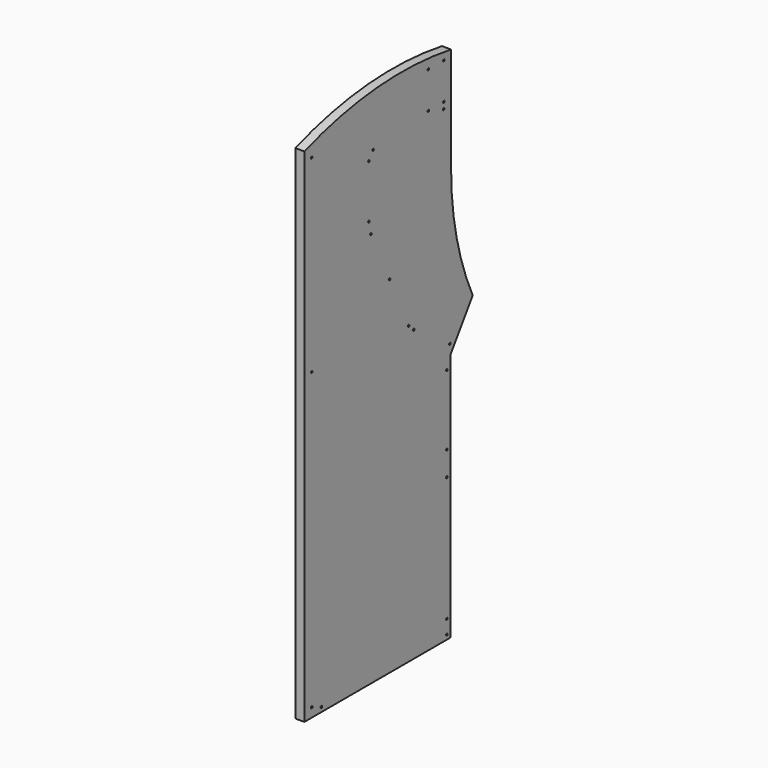
from build123d import *

# Parameters (mm, degrees)
F1_DEPTH       = 30
F2_D           = 6.6
F2_CSINK_D     = 13.44
F2_CSINK_ANGLE = 90


# Not quite as in the source:
# - a feature names something its author has since deleted; it is built from what else it names


with BuildPart() as f1:
    # F0 (on Right) → F1 (new body)
    with BuildSketch(Plane.YZ):
        with BuildLine():
            Line((-278.9958539005, 831.5081800917), (-278.9958539005, -818.4918199083))
            Line((-278.9958539005, -818.4918199083), (321.0041460995, -818.4918199083))
            Line((321.0041460995, -818.4918199083), (321.0041460995, 0))
            Line((321.0041460995, 0), (412.2409460549, 134.0160220861))
            ThreePointArc((412.2409460549, 134.0160220861), (346.0454150195, 328.1386194333), (323.6229111026, 532.0078482247))
            Line((323.6229111026, 532.0078482247), (323.6229111026, 881.5081800917))
            ThreePointArc((323.6229111026, 881.5081800917), (19.1314569656, 894.8597016737), (-278.9958539005, 831.5081800917))
        make_face()
    extrude(amount=F1_DEPTH)

    # F2 (through all)
    with Locations(Plane(origin=(0, 0, 0), x_dir=(0, 1, 0), z_dir=(-1, 0, 0))):
        with Locations((293.6229111026, -742.0078482247), (293.6229111026, -862.0078482247), (229.6229111026, -862.0078482247), (229.6229111026, -742.0078482247), (-248.9958539005, -801.5081800917), (-248.9958539005, -181.5081800917), (306.0041460995, 38.4918199083), (306.0041460995, 348.4918199083), (306.0041460995, 758.4918199083), (306.0041460995, 803.4918199083), (-208.9958539005, 803.4918199083), (-248.9958539005, 788.4918199083), (306.0041460995, 268.4918199083), (318.5190369661, -31.8890116707), (169.7269624564, -133.1852039145), (149.0127494203, -152.9318064879), (70.5869059911, -319.3811593927), (-5.7078003883, -481.3074320555), (-13.9958539005, -520.7695364952), (-13.9958539005, -695.7695364952), (293.033330664, -721.4207649231), (3.033330664, -721.4207649231)):
            CounterSinkHole(F2_D / 2, F2_CSINK_D / 2, counter_sink_angle=F2_CSINK_ANGLE)


solid = f1.part
